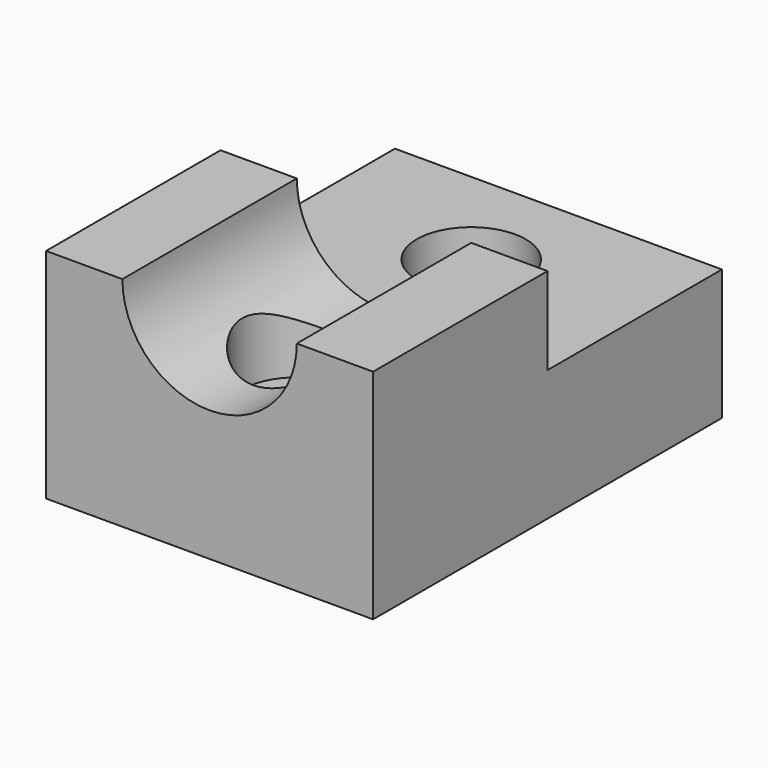
from build123d import *

# Parameters (mm, degrees)
F0_W           = 30
F0_H           = 40
F1_DEPTH       = 20
F7_D           = 5
F7_CBORE_D     = 10
F7_CBORE_DEPTH = 12
F8_DEPTH       = 40
F4_DEPTH       = 20


with BuildPart() as f1:
    # F0 (on Top) → F1 (new body)
    with BuildSketch(Plane.XY):
        Rectangle(F0_W, F0_H)
    extrude(amount=F1_DEPTH)

    # F7 (through all)
    with Locations(Plane.XY.offset(20)):
        with Locations((0, -10), (0, 10)):
            CounterBoreHole(F7_D / 2, F7_CBORE_D / 2, F7_CBORE_DEPTH)

    # F6 (on face) → F8 (cut)
    with BuildSketch(Plane.XZ.offset(20)):
        with BuildLine():
            ThreePointArc((-8, 20), (0, 12), (8, 20))
            Line((8, 20), (-8, 20))
        make_face()
        with BuildLine():
            Line((-8, 20), (8, 20))
            ThreePointArc((8, 20), (0, 28), (-8, 20))
        make_face()
    extrude(amount=-F8_DEPTH, mode=Mode.SUBTRACT)

    # F3 (on face) → F4 (cut)
    with BuildSketch(Plane(origin=(0, 20, 0), x_dir=(-1, 0, 0), z_dir=(0, 1, 0))):
        with BuildLine():
            ThreePointArc((8, 20), (5.6568542495, 14.3431457505), (0, 12))
            Line((0, 12), (15, 12))
            Line((15, 12), (15, 20))
            Line((15, 20), (8, 20))
        make_face()
        with BuildLine():
            Line((-15, 12), (0, 12))
            ThreePointArc((0, 12), (-5.6568542495, 14.3431457505), (-8, 20))
            Line((-8, 20), (-15, 20))
            Line((-15, 20), (-15, 12))
        make_face()
    extrude(amount=-F4_DEPTH, mode=Mode.SUBTRACT)


solid = f1.part
